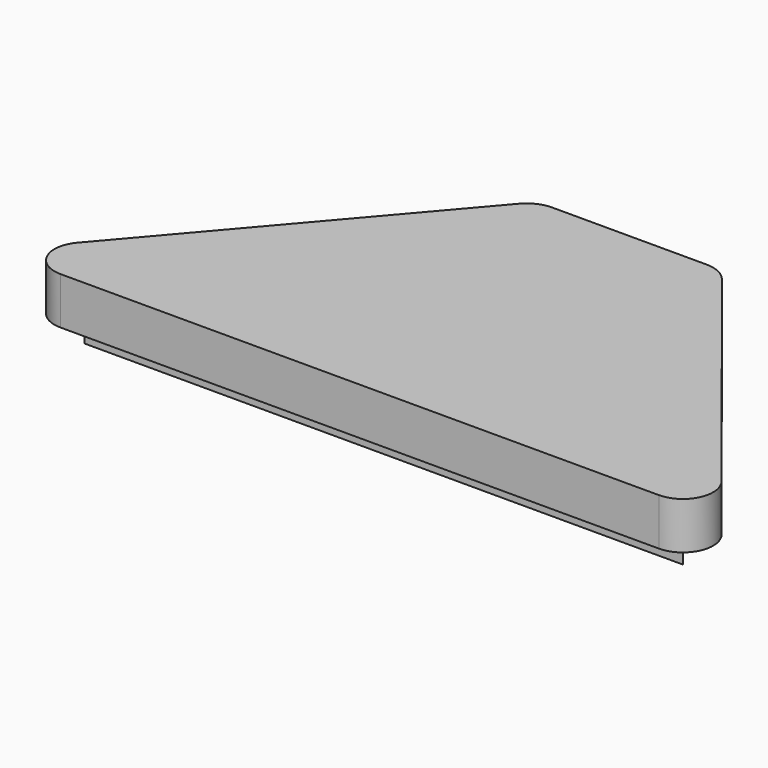
from build123d import *

# Parameters (mm, degrees)
F0_TEXT_SIZE = 9.0532412564
F1_DEPTH     = 3.175
F2_DEPTH     = 1.778


# Not quite as in the source:
# - Text() gives the source's letters only with a copy of the font that has no kerning and outlines rounded to 1/6400 em; it was checked with that copy


with BuildPart() as f1:
    # F0 (on Top) → F1 (new body)
    with BuildSketch(Plane.XY):
        with BuildLine():
            ThreePointArc((55.9706334899, 10.2677550296), (55.2196628561, 10.8660220358), (54.2835542571, 11.0795190955))
            Line((54.2835542571, 11.0795190955), (43.8744305403, 11.0795190955))
            ThreePointArc((43.8744305403, 11.0795190955), (42.9708956166, 10.8813621901), (42.2332168156, 10.3232658688))
            Line((42.2332168156, 10.3232658688), (26.8459523442, -7.6798335628))
            ThreePointArc((26.8459523442, -7.6798335628), (26.5451247019, -9.8504516305), (28.3906240851, -11.03206582))
            Line((28.3906240851, -11.03206582), (68.7567624406, -11.03206582))
            ThreePointArc((68.7567624406, -11.03206582), (70.5878240315, -9.8811092073), (70.3446017185, -7.7320790585))
            Line((70.3446017185, -7.7320790585), (55.9706334899, 10.2677550296))
        make_face()
        Polygon((53.3734038081, 6.5065571233), (52.6622038081, 6.5065571233), (52.6622038081, 4.75826582), (53.2921092479, 4.75826582), (54.5500487986, -2.8146303046), (59.1906283424, 2.9791471498), (68.7567624406, -9.00006582), (28.3906240851, -9.00006582), (42.2482038081, 7.2133024559), (47.5120069422, 1.054652789), (48.1198047589, 4.75826582), (48.7506038081, 4.75826582), (48.7506038081, 6.5065571233), (48.0394038081, 6.5065571233), (48.0394038081, 7.8946619317), (50.7057806615, 9.0475190955), (53.3734038081, 7.9009105085), align=None, mode=Mode.SUBTRACT)
        Polygon((52.6622038081, 4.75826582), (52.6622038081, 6.5065571233), (53.3734038081, 6.5065571233), (53.3734038081, 7.9009105085), (50.7057806615, 9.0475190955), (48.0394038081, 7.8946619317), (48.0394038081, 6.5065571233), (48.7506038081, 6.5065571233), (48.7506038081, 4.75826582), (48.1198047589, 4.75826582), (47.5120069422, 1.054652789), (42.2482038081, 7.2133024559), (28.3906240851, -9.00006582), (68.7567624406, -9.00006582), (59.1906283424, 2.9791471498), (54.5500487986, -2.8146303046), (53.2921092479, 4.75826582), align=None)
        Polygon((52.7718016898, -6.7412436176), (59.1893792737, 1.2711212102), (66.5396451756, -7.93326582), (30.7057835311, -7.93326582), (42.2482038081, 5.5713659041), align=None, mode=Mode.SUBTRACT)
        Polygon((49.8174038081, 7.5011675847), (50.7070269546, 7.8858125445), (51.5954038081, 7.5039668067), (51.5954038081, 3.69146582), (52.3878983683, 3.69146582), (53.6543829126, -3.932871845), (52.7451199276, -5.068089404), (48.4189387818, -0.0064574634), (49.0258028573, 3.69146582), (49.8174038081, 3.69146582), align=None, mode=Mode.SUBTRACT)
        Polygon((66.5396451756, -7.93326582), (59.1893792737, 1.2711212102), (52.7718016898, -6.7412436176), (42.2482038081, 5.5713659041), (30.7057835311, -7.93326582), align=None)
        with BuildLine():
            Line((37.2903708137, -7.4353703988), (37.2903708137, -0.9722048831))
            Line((37.2903708137, -0.9722048831), (39.3018878554, -0.9722048831))
            add(Edge.make_bspline(
                [(39.3018878554, -0.9722048831), (40.6768488712, -0.9722048831), (41.2978446386, -1.3633331968)],
                knots=[0, 0, 0, 1, 1, 1], degree=2))
            add(Edge.make_bspline(
                [(41.2978446386, -1.3633331968), (41.918840406, -1.7544615104), (41.918840406, -2.607446585)],
                knots=[0, 0, 0, 1, 1, 1], degree=2))
            add(Edge.make_bspline(
                [(41.918840406, -2.607446585), (41.918840406, -3.187419853), (41.6472431684, -3.5587442014)],
                knots=[0, 0, 0, 1, 1, 1], degree=2))
            add(Edge.make_bspline(
                [(41.6472431684, -3.5587442014), (41.3756459307, -3.9300685499), (40.9243984368, -4.005040704)],
                knots=[0, 0, 0, 1, 1, 1], degree=2))
            Line((40.9243984368, -4.005040704), (40.9243984368, -4.0488923413))
            add(Edge.make_bspline(
                [(40.9243984368, -4.0488923413), (41.5383213595, -4.1861055291), (41.8106258817, -4.5616735844)],
                knots=[0, 0, 0, 1, 1, 1], degree=2))
            add(Edge.make_bspline(
                [(41.8106258817, -4.5616735844), (42.0829304038, -4.9372416396), (42.0829304038, -5.561066545)],
                knots=[0, 0, 0, 1, 1, 1], degree=2))
            add(Edge.make_bspline(
                [(42.0829304038, -5.561066545), (42.0829304038, -6.4451721364), (41.4435452401, -6.9402712676)],
                knots=[0, 0, 0, 1, 1, 1], degree=2))
            add(Edge.make_bspline(
                [(41.4435452401, -6.9402712676), (40.8041600764, -7.4353703988), (39.707869143, -7.4353703988)],
                knots=[0, 0, 0, 1, 1, 1], degree=2))
            Line((39.707869143, -7.4353703988), (37.2903708137, -7.4353703988))
        make_face(mode=Mode.SUBTRACT)
        with BuildLine():
            add(Edge.make_bspline(
                [(47.8600299806, -1.8075078459), (48.7356481583, -2.6428108087), (48.7356481583, -4.1422538918)],
                knots=[0, 0, 0, 1, 1, 1], degree=2))
            add(Edge.make_bspline(
                [(48.7356481583, -4.1422538918), (48.7356481583, -5.7378876632), (47.8267876103, -6.586629031)],
                knots=[0, 0, 0, 1, 1, 1], degree=2))
            add(Edge.make_bspline(
                [(47.8267876103, -6.586629031), (46.9179270623, -7.4353703988), (45.2034694994, -7.4353703988)],
                knots=[0, 0, 0, 1, 1, 1], degree=2))
            Line((45.2034694994, -7.4353703988), (43.3730172829, -7.4353703988))
            Line((43.3730172829, -7.4353703988), (43.3730172829, -0.9722048831))
            Line((43.3730172829, -0.9722048831), (45.4015091519, -0.9722048831))
            add(Edge.make_bspline(
                [(45.4015091519, -0.9722048831), (46.9844118028, -0.9722048831), (47.8600299806, -1.8075078459)],
                knots=[0, 0, 0, 1, 1, 1], degree=2))
        make_face(mode=Mode.SUBTRACT)
        Polygon((51.5954038081, 7.5039668067), (50.7070269546, 7.8858125445), (49.8174038081, 7.5011675847), (49.8174038081, 3.69146582), (49.0258028573, 3.69146582), (48.4189387818, -0.0064574634), (52.7451199276, -5.068089404), (53.6543829126, -3.932871845), (52.3878983683, 3.69146582), (51.5954038081, 3.69146582), align=None)
        with Locations((36.4769936696, -7.4353703988)):
            Text('BD', F0_TEXT_SIZE, font='Open Sans', font_style=FontStyle.BOLD, text_align=(TextAlign.LEFT, TextAlign.BOTTOM))
        with BuildLine():
            add(Edge.make_bspline(
                [(45.3307807046, -6.3037152418), (47.3111772294, -6.3037152418), (47.3111772294, -4.1776181155)],
                knots=[0, 0, 0, 1, 1, 1], degree=2))
            add(Edge.make_bspline(
                [(47.3111772294, -4.1776181155), (47.3111772294, -2.0953726265), (45.4722375992, -2.0953726265)],
                knots=[0, 0, 0, 1, 1, 1], degree=2))
            Line((45.4722375992, -2.0953726265), (44.7437345918, -2.0953726265))
            Line((44.7437345918, -2.0953726265), (44.7437345918, -6.3037152418))
            Line((44.7437345918, -6.3037152418), (45.3307807046, -6.3037152418))
        make_face()
        with BuildLine():
            Line((39.5098294905, -4.6189636267), (38.6610881227, -4.6189636267))
            Line((38.6610881227, -4.6189636267), (38.6610881227, -6.3037152418))
            Line((38.6610881227, -6.3037152418), (39.5536811278, -6.3037152418))
            add(Edge.make_bspline(
                [(39.5536811278, -6.3037152418), (40.1195087063, -6.3037152418), (40.3889840906, -6.087286193)],
                knots=[0, 0, 0, 1, 1, 1], degree=2))
            add(Edge.make_bspline(
                [(40.3889840906, -6.087286193), (40.6584594749, -5.8708571442), (40.6584594749, -5.4238533572)],
                knots=[0, 0, 0, 1, 1, 1], degree=2))
            add(Edge.make_bspline(
                [(40.6584594749, -5.4238533572), (40.6584594749, -4.6189636267), (39.5098294905, -4.6189636267)],
                knots=[0, 0, 0, 1, 1, 1], degree=2))
        make_face()
        with BuildLine():
            Line((38.6610881227, -2.0953726265), (38.6610881227, -3.5325746759))
            Line((38.6610881227, -3.5325746759), (39.4560758705, -3.5325746759))
            add(Edge.make_bspline(
                [(39.4560758705, -3.5325746759), (40.0134160354, -3.5325746759), (40.2630874544, -3.3599972645)],
                knots=[0, 0, 0, 1, 1, 1], degree=2))
            add(Edge.make_bspline(
                [(40.2630874544, -3.3599972645), (40.5127588734, -3.187419853), (40.5127588734, -2.7899259791)],
                knots=[0, 0, 0, 1, 1, 1], degree=2))
            add(Edge.make_bspline(
                [(40.5127588734, -2.7899259791), (40.5127588734, -2.4178943462), (40.2411616357, -2.2566334864)],
                knots=[0, 0, 0, 1, 1, 1], degree=2))
            add(Edge.make_bspline(
                [(40.2411616357, -2.2566334864), (39.969564398, -2.0953726265), (39.3811037164, -2.0953726265)],
                knots=[0, 0, 0, 1, 1, 1], degree=2))
            Line((39.3811037164, -2.0953726265), (38.6610881227, -2.0953726265))
        make_face()
    extrude(amount=F1_DEPTH)

    # F0 (on Top) → F2 (join)
    with BuildSketch(Plane.XY):
        Polygon((52.6622038081, 4.75826582), (52.6622038081, 6.5065571233), (53.3734038081, 6.5065571233), (53.3734038081, 7.9009105085), (50.7057806615, 9.0475190955), (48.0394038081, 7.8946619317), (48.0394038081, 6.5065571233), (48.7506038081, 6.5065571233), (48.7506038081, 4.75826582), (48.1198047589, 4.75826582), (47.5120069422, 1.054652789), (42.2482038081, 7.2133024559), (28.3906240851, -9.00006582), (68.7567624406, -9.00006582), (59.1906283424, 2.9791471498), (54.5500487986, -2.8146303046), (53.2921092479, 4.75826582), align=None)
        Polygon((52.7718016898, -6.7412436176), (59.1893792737, 1.2711212102), (66.5396451756, -7.93326582), (30.7057835311, -7.93326582), (42.2482038081, 5.5713659041), align=None, mode=Mode.SUBTRACT)
        Polygon((49.8174038081, 7.5011675847), (50.7070269546, 7.8858125445), (51.5954038081, 7.5039668067), (51.5954038081, 3.69146582), (52.3878983683, 3.69146582), (53.6543829126, -3.932871845), (52.7451199276, -5.068089404), (48.4189387818, -0.0064574634), (49.0258028573, 3.69146582), (49.8174038081, 3.69146582), align=None, mode=Mode.SUBTRACT)
        with Locations((36.4769936696, -7.4353703988)):
            Text('BD', F0_TEXT_SIZE, font='Open Sans', font_style=FontStyle.BOLD, text_align=(TextAlign.LEFT, TextAlign.BOTTOM))
    extrude(amount=-F2_DEPTH)


solid = f1.part
